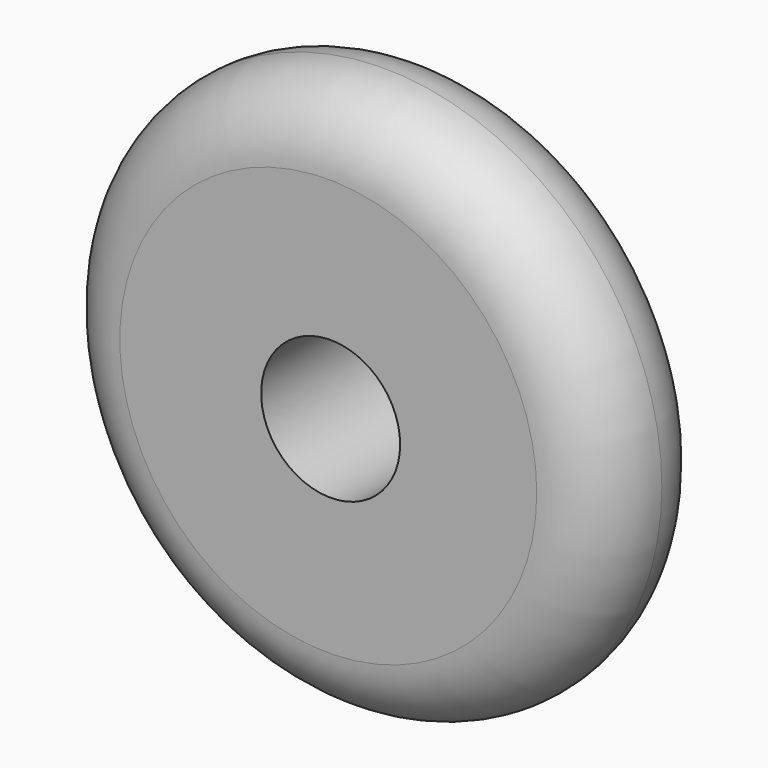
from build123d import *

# Parameters (mm, degrees)
F0_R     = 50.8
F0_R_2   = 25.4
F0_R_3   = 12.7
F1_DEPTH = 12.7
F2_R     = 12.69999


# Not quite as in the source:
# - a fillet or chamfer is up to 0.001 mm smaller than in the source, because OpenCascade refuses the exact size


with BuildPart() as f1:
    # F0 (on Front) → F1 (new body, symmetric)
    with BuildSketch(Plane.XZ):
        with Locations((-0.4342335526, 0.3162413696)):
            Circle(F0_R)
        Circle(F0_R_2, mode=Mode.SUBTRACT)
        Circle(F0_R_2)
        Circle(F0_R_3, mode=Mode.SUBTRACT)
    extrude(amount=F1_DEPTH, both=True)

    # F2 (radius 12.7 in the source; OpenCascade refuses exactly that, so slightly less here)
    f2_edges = [f1.edges().sort_by_distance(p)[0] for p in [
        (-51.234234, 12.7, 0.316241),
        (-51.234234, -12.7, 0.316241),
    ]]
    fillet(f2_edges, radius=F2_R)


solid = f1.part
